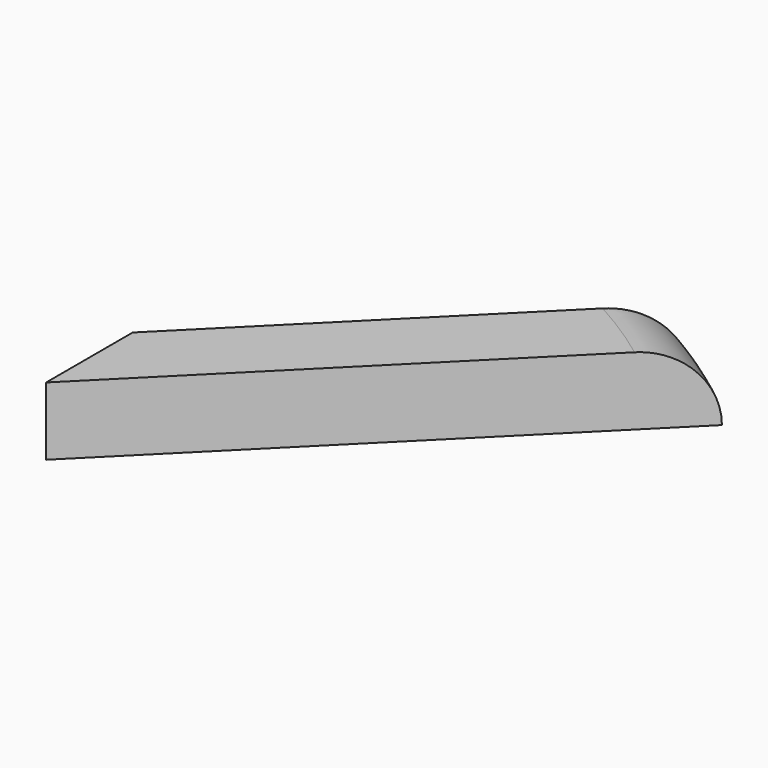
from build123d import *

# Parameters (mm, degrees)
F2_DEPTH = 25.4
F3_R     = 25.39999


# Not quite as in the source:
# - a fillet or chamfer is up to 0.001 mm smaller than in the source, because OpenCascade refuses the exact size


with BuildPart() as f2:
    # F1 (on face) → F2 (new body)
    with BuildSketch(Plane.XY):
        with BuildLine():
            Line((0, 80.8223050896), (0, 40.4111525448))
            Line((0, 40.4111525448), (140.1712134682, 180.582366013))
            ThreePointArc((140.1712134682, 180.582366013), (128.3961041965, 189.1359310844), (116.1005682623, 196.9228733519))
            Line((116.1005682623, 196.9228733519), (0, 80.8223050896))
        make_face()
    extrude(amount=F2_DEPTH)

    # F3 (radius 25.4 in the source; OpenCascade refuses exactly that, so slightly less here)
    f3_edges = [f2.edges().sort_by_distance(p)[0] for p in [
        (128.396104, 189.135931, 25.4),
    ]]
    fillet(f3_edges, radius=F3_R)


solid = f2.part
